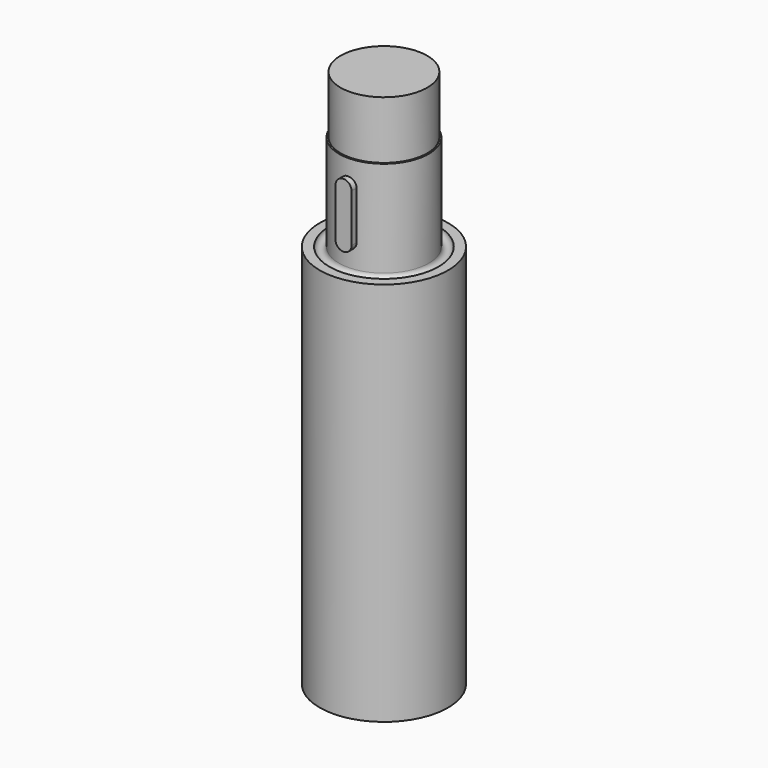
from build123d import *

# Parameters (mm, degrees)
F0_W          = 13.5
F0_H          = 18
F4_DEPTH      = 1.75
F4_DEPTH_BACK = 5


with BuildPart() as f1:
    # F0 (on Front) → F1 (revolve)
    with BuildSketch(Plane.XZ):
        with BuildLine():
            Line((0, -120), (0, 30))
            Line((0, 30), (-13.5, 30))
            Line((-13.5, 30), (-14, 30))
            Line((-14, 30), (-14, 0))
            ThreePointArc((-14, 0), (-15.5, -1.5), (-17, 0))
            Line((-17, 0), (-20, 0))
            Line((-20, 0), (-20, -120))
            Line((-20, -120), (0, -120))
        make_face()
        with Locations((-6.75, 39)):
            Rectangle(F0_W, F0_H)
    revolve(axis=Axis((0, 0, -45), (0, 0, -1)))


with BuildPart() as f4:
    # F3 (on offset) → F4 (new body, two sides)
    with BuildSketch(Plane.XZ.offset(14)) as f4_sk:
        with BuildLine():
            Line((0, 25), (0, 22.5))
            Line((0, 22.5), (0, 20))
            ThreePointArc((0, 20), (1.767766953, 20.732233047), (2.5, 22.5))
            ThreePointArc((2.5, 22.5), (1.767766953, 24.267766953), (0, 25))
        make_face()
        with BuildLine():
            Line((0, 20), (0, 22.5))
            Line((0, 22.5), (0, 25))
            ThreePointArc((0, 25), (-1.767766953, 24.267766953), (-2.5, 22.5))
            ThreePointArc((-2.5, 22.5), (-1.767766953, 20.732233047), (0, 20))
        make_face()
        with BuildLine():
            ThreePointArc((2.5, 22.5), (1.767766953, 20.732233047), (0, 20))
            Line((0, 20), (0, 10))
            ThreePointArc((0, 10), (1.767766953, 9.267766953), (2.5, 7.5))
            Line((2.5, 7.5), (2.5, 22.5))
        make_face()
        with BuildLine():
            Line((0, 10), (0, 20))
            ThreePointArc((0, 20), (-1.767766953, 20.732233047), (-2.5, 22.5))
            Line((-2.5, 22.5), (-2.5, 7.5))
            ThreePointArc((-2.5, 7.5), (-1.767766953, 9.267766953), (0, 10))
        make_face()
        with BuildLine():
            ThreePointArc((2.5, 7.5), (1.767766953, 9.267766953), (0, 10))
            Line((0, 10), (0, 7.5))
            Line((0, 7.5), (0, 5))
            ThreePointArc((0, 5), (1.767766953, 5.732233047), (2.5, 7.5))
        make_face()
        with BuildLine():
            Line((0, 7.5), (0, 10))
            ThreePointArc((0, 10), (-1.767766953, 9.267766953), (-2.5, 7.5))
            ThreePointArc((-2.5, 7.5), (-1.767766953, 5.732233047), (0, 5))
            Line((0, 5), (0, 7.5))
        make_face()
    extrude(amount=F4_DEPTH)
    extrude(f4_sk.sketch, amount=-F4_DEPTH_BACK)


solid = Compound([f1.part, f4.part])
